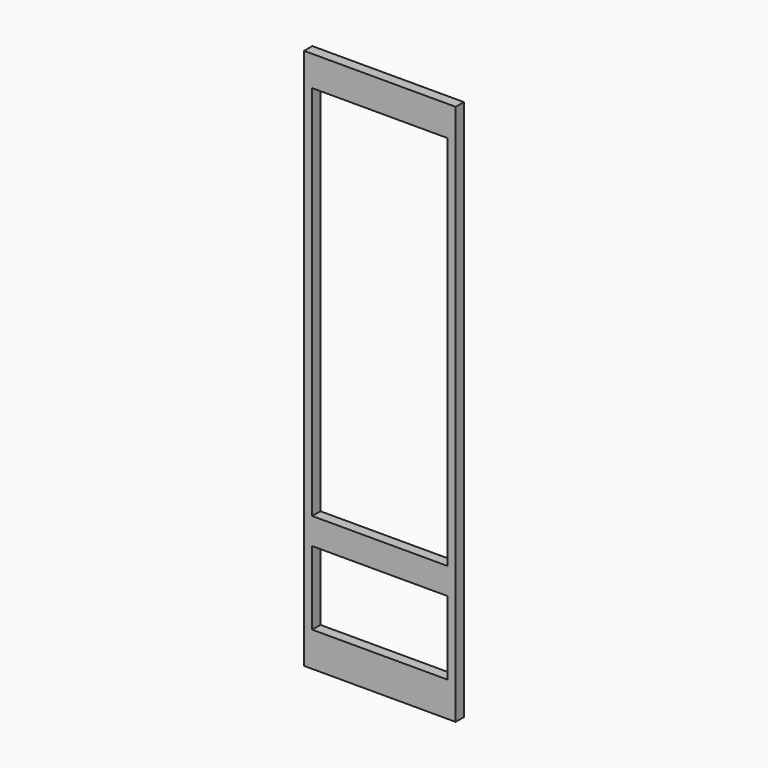
from build123d import *

# Parameters (mm, degrees)
F0_W          = 654.05
F0_H          = 2413
F0_W_2        = 584.2
F0_H_2        = 317.5
F0_H_3        = 1625.6
F1_DEPTH      = 22.225
F1_DEPTH_BACK = 22.225
F2_W          = 1248.5843106929
F2_H          = 271.0993243682
F2_H_2        = 504.0157202398
F3_DEPTH      = 22.226
F3_DEPTH_BACK = 22.226


# Not quite as in the source:
# - a length typed as a fraction of an inch, garbled in the dataset ("3 / 203.2 mm" for 3/8 in), is restored


with BuildPart() as f1:
    # F0 (on Front) → F1 (new body, two sides)
    with BuildSketch(Plane.XZ) as f1_sk:
        Rectangle(F0_W, F0_H)
        with Locations((0, -822.325)):
            Rectangle(F0_W_2, F0_H_2, mode=Mode.SUBTRACT)
        with Locations((0, 263.525)):
            Rectangle(F0_W_2, F0_H_3, mode=Mode.SUBTRACT)
    extrude(amount=F1_DEPTH)
    extrude(f1_sk.sketch, amount=-F1_DEPTH_BACK)

    # F2 (on Front) → F3 (cut, two sides)
    with BuildSketch(Plane.XZ) as f3_sk:
        with Locations((62.8663003445, 1342.0496621841)):
            Rectangle(F2_W, F2_H)
        with Locations((62.8663003445, -1382.3078601199)):
            Rectangle(F2_W, F2_H_2)
    extrude(amount=-F3_DEPTH, mode=Mode.SUBTRACT)
    extrude(f3_sk.sketch, amount=F3_DEPTH_BACK, mode=Mode.SUBTRACT)


solid = f1.part
